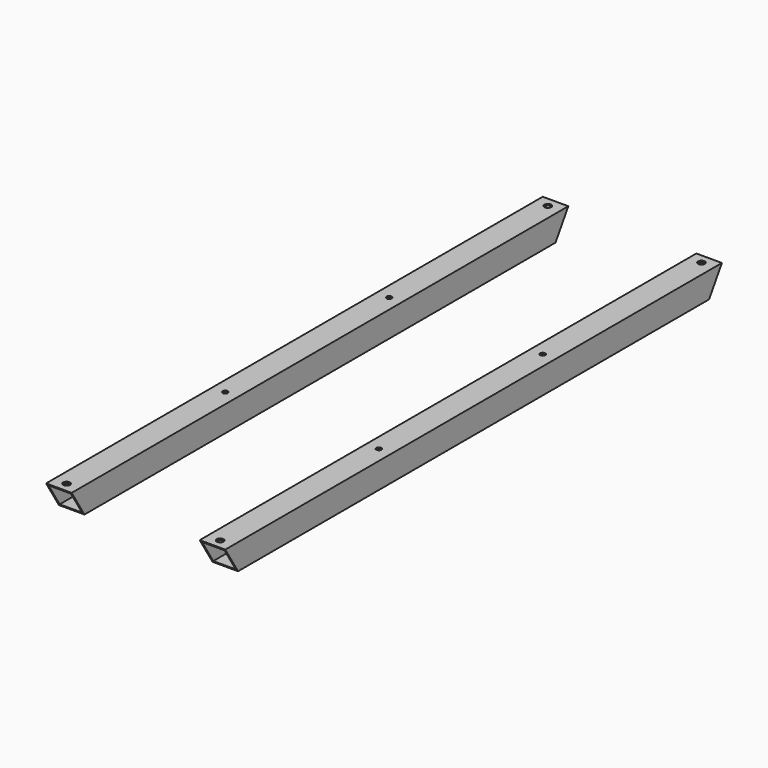
from build123d import *

# Parameters (mm, degrees)
F0_W     = 25.4
F0_H     = 25.4
F0_W_2   = 22.225
F0_H_2   = 22.225
F1_DEPTH = 615.95
F3_D     = 5.1054
F5_DEPTH = 25.4
F7_D     = 12.7
F7_DEPTH = 1.5875
F7_TIP   = 3.8154649308
F9_D     = 6.7564


# Not quite as in the source:
# - a length typed as a fraction of an inch, garbled in the dataset ("3 / 203.2 mm" for 3/8 in), is restored
# - a feature names something its author has since deleted; it is built from what else it names


with BuildPart() as f1:
    # F0 (on Front) → F1 (new body)
    with BuildSketch(Plane.XZ):
        with Locations((76.2, 12.7)):
            Rectangle(F0_W, F0_H)
        with Locations((76.2, 12.7)):
            Rectangle(F0_W_2, F0_H_2, mode=Mode.SUBTRACT)
    extrude(amount=F1_DEPTH)

    # F3 (through all)
    with Locations(Plane.XY.offset(25.4)):
        with Locations((76.2, -206.375), (76.2, -409.575)):
            Hole(F3_D / 2)

    # F4 (on face) → F5 (cut)
    with BuildSketch(Plane.YZ.offset(88.9)):
        Polygon((0, 0), (0, 25.4), (-15.875, 0), align=None)
        Polygon((-600.075, 0), (-615.95, 25.4), (-615.95, 0), align=None)
    extrude(amount=-F5_DEPTH, mode=Mode.SUBTRACT)

    # F7
    with Locations(Plane(origin=(0, 0, 0), x_dir=(1, 0, 0), z_dir=(0, 0, -1))):
        with Locations((76.2, 409.575), (76.2, 206.375)):
            Hole(F7_D / 2, depth=F7_DEPTH)
            with Locations((0, 0, -(F7_DEPTH + F7_TIP / 2))):  # 118° drill point
                Cone(0, F7_D / 2, F7_TIP, mode=Mode.SUBTRACT)

    # F9 (through all)
    with Locations(Plane.XY.offset(25.4)):
        with Locations((76.2, -606.425), (76.2, -9.525)):
            Hole(F9_D / 2)


with BuildPart() as f10_1:
    # F10: instance of F1
    add(f1.part.mirror(Plane.YZ))


solid = Compound([f1.part, f10_1.part])
